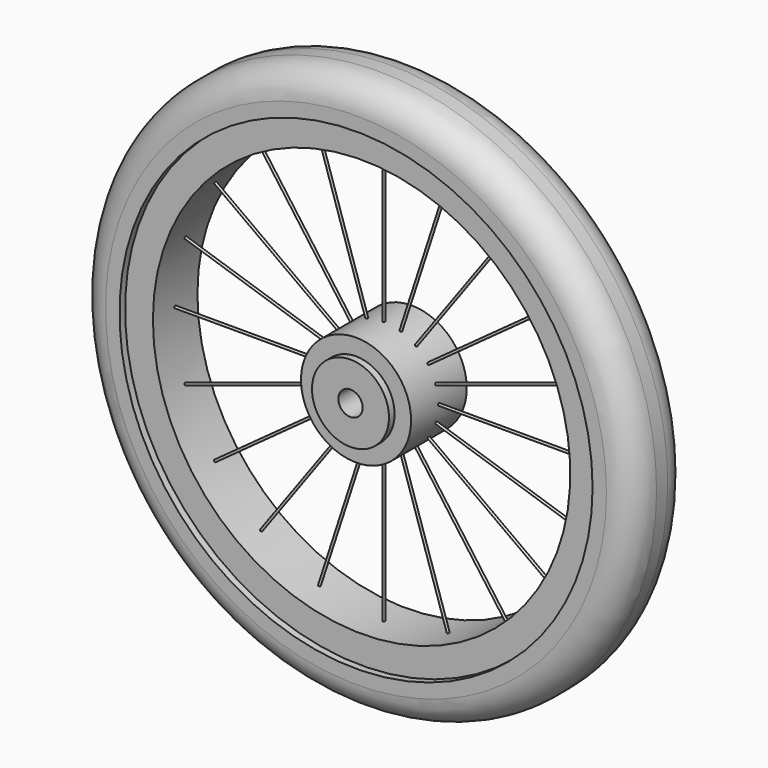
from build123d import *

# Parameters (mm, degrees)
F0_R          = 35.1337076678
F0_R_2        = 11.0975726691
F1_DEPTH      = 38.1
F2_DEPTH      = 31.75
F0_R_3        = 215.9
F3_DEPTH      = 25.4
F7_END_RADIUS = 190.5
F6_R          = 1.0573561201
F7_REACH      = 168.6504547306
F8_COUNT      = 20
F8_ANGLE      = 342
F0_R_4        = 254
F9_DEPTH      = 31.75
F10_R         = 25.4


with BuildPart() as f1:
    # F0 (on Front) → F1 (new body, symmetric)
    with BuildSketch(Plane.XZ):
        Circle(F0_R)
        Circle(F0_R_2, mode=Mode.SUBTRACT)
    extrude(amount=F1_DEPTH, both=True)

    # F0 (on Front) → F2 (join, symmetric)
    with BuildSketch(Plane.XZ):
        with BuildLine():
            ThreePointArc((-50.2431450113, 0), (0, -50.2431450113), (50.2431450113, 0))
            ThreePointArc((50.2431450113, 0), (0, 50.2431450113), (-50.2431450113, 0))
        make_face()
        Circle(F0_R, mode=Mode.SUBTRACT)
    extrude(amount=F2_DEPTH, both=True)


with BuildPart() as f3:
    # F0 (on Front) → F3 (new body, symmetric)
    with BuildSketch(Plane.XZ):
        Circle(F0_R_3)
        with BuildLine():
            ThreePointArc((190.5, 0), (0, -190.5), (-190.5, 0))
            ThreePointArc((-190.5, 0), (0, 190.5), (190.5, 0))
        make_face(mode=Mode.SUBTRACT)
    extrude(amount=F3_DEPTH, both=True)


with BuildPart() as f7:
    f7_end = (Plane.ZX.offset(-12.7) * Cylinder(F7_END_RADIUS, 1568.087519723, mode=Mode.PRIVATE)).faces().sort_by_distance((0, -12.7, 190.5))[0]
    # F6 (on offset) → F7 (new body, up to the whole of a round face its end follows)
    with BuildSketch(Plane.YZ.offset(-50.2412)):
        Circle(F6_R)
    f7_long = extrude(amount=-F7_REACH, mode=Mode.PRIVATE)
    add(split(f7_long, bisect_by=f7_end, keep=Keep.BOTTOM, mode=Mode.PRIVATE))


with BuildPart() as f8_1:
    # F8: instance of F7
    add(f7.part.rotate(Axis((0, -0.9538419545, 0), (0, -1, 0)), 1 * F8_ANGLE / (F8_COUNT - 1)))


with BuildPart() as f8_2:
    # F8: instance of F7
    add(f7.part.rotate(Axis((0, -0.9538419545, 0), (0, -1, 0)), 2 * F8_ANGLE / (F8_COUNT - 1)))


with BuildPart() as f8_3:
    # F8: instance of F7
    add(f7.part.rotate(Axis((0, -0.9538419545, 0), (0, -1, 0)), 3 * F8_ANGLE / (F8_COUNT - 1)))


with BuildPart() as f8_4:
    # F8: instance of F7
    add(f7.part.rotate(Axis((0, -0.9538419545, 0), (0, -1, 0)), 4 * F8_ANGLE / (F8_COUNT - 1)))


with BuildPart() as f8_5:
    # F8: instance of F7
    add(f7.part.rotate(Axis((0, -0.9538419545, 0), (0, -1, 0)), 5 * F8_ANGLE / (F8_COUNT - 1)))


with BuildPart() as f8_6:
    # F8: instance of F7
    add(f7.part.rotate(Axis((0, -0.9538419545, 0), (0, -1, 0)), 6 * F8_ANGLE / (F8_COUNT - 1)))


with BuildPart() as f8_7:
    # F8: instance of F7
    add(f7.part.rotate(Axis((0, -0.9538419545, 0), (0, -1, 0)), 7 * F8_ANGLE / (F8_COUNT - 1)))


with BuildPart() as f8_8:
    # F8: instance of F7
    add(f7.part.rotate(Axis((0, -0.9538419545, 0), (0, -1, 0)), 8 * F8_ANGLE / (F8_COUNT - 1)))


with BuildPart() as f8_9:
    # F8: instance of F7
    add(f7.part.rotate(Axis((0, -0.9538419545, 0), (0, -1, 0)), 9 * F8_ANGLE / (F8_COUNT - 1)))


with BuildPart() as f8_10:
    # F8: instance of F7
    add(f7.part.rotate(Axis((0, -0.9538419545, 0), (0, -1, 0)), 10 * F8_ANGLE / (F8_COUNT - 1)))


with BuildPart() as f8_11:
    # F8: instance of F7
    add(f7.part.rotate(Axis((0, -0.9538419545, 0), (0, -1, 0)), 11 * F8_ANGLE / (F8_COUNT - 1)))


with BuildPart() as f8_12:
    # F8: instance of F7
    add(f7.part.rotate(Axis((0, -0.9538419545, 0), (0, -1, 0)), 12 * F8_ANGLE / (F8_COUNT - 1)))


with BuildPart() as f8_13:
    # F8: instance of F7
    add(f7.part.rotate(Axis((0, -0.9538419545, 0), (0, -1, 0)), 13 * F8_ANGLE / (F8_COUNT - 1)))


with BuildPart() as f8_14:
    # F8: instance of F7
    add(f7.part.rotate(Axis((0, -0.9538419545, 0), (0, -1, 0)), 14 * F8_ANGLE / (F8_COUNT - 1)))


with BuildPart() as f8_15:
    # F8: instance of F7
    add(f7.part.rotate(Axis((0, -0.9538419545, 0), (0, -1, 0)), 15 * F8_ANGLE / (F8_COUNT - 1)))


with BuildPart() as f8_16:
    # F8: instance of F7
    add(f7.part.rotate(Axis((0, -0.9538419545, 0), (0, -1, 0)), 16 * F8_ANGLE / (F8_COUNT - 1)))


with BuildPart() as f8_17:
    # F8: instance of F7
    add(f7.part.rotate(Axis((0, -0.9538419545, 0), (0, -1, 0)), 17 * F8_ANGLE / (F8_COUNT - 1)))


with BuildPart() as f8_18:
    # F8: instance of F7
    add(f7.part.rotate(Axis((0, -0.9538419545, 0), (0, -1, 0)), 18 * F8_ANGLE / (F8_COUNT - 1)))


with BuildPart() as f8_19:
    # F8: instance of F7
    add(f7.part.rotate(Axis((0, -0.9538419545, 0), (0, -1, 0)), 19 * F8_ANGLE / (F8_COUNT - 1)))


with BuildPart() as f9:
    # F0 (on Front) → F9 (new body, symmetric)
    with BuildSketch(Plane.XZ):
        Circle(F0_R_4)
        Circle(F0_R_3, mode=Mode.SUBTRACT)
    extrude(amount=F9_DEPTH, both=True)

    # F10
    f10_edges = [f9.edges().sort_by_distance(p)[0] for p in [
        (-254, 31.75, 0),
        (-254, -31.75, 0),
    ]]
    fillet(f10_edges, radius=F10_R)


solid = Compound([f1.part, f3.part, f7.part, f8_1.part, f8_2.part, f8_3.part, f8_4.part, f8_5.part, f8_6.part, f8_7.part, f8_8.part, f8_9.part, f8_10.part, f8_11.part, f8_12.part, f8_13.part, f8_14.part, f8_15.part, f8_16.part, f8_17.part, f8_18.part, f8_19.part, f9.part])
